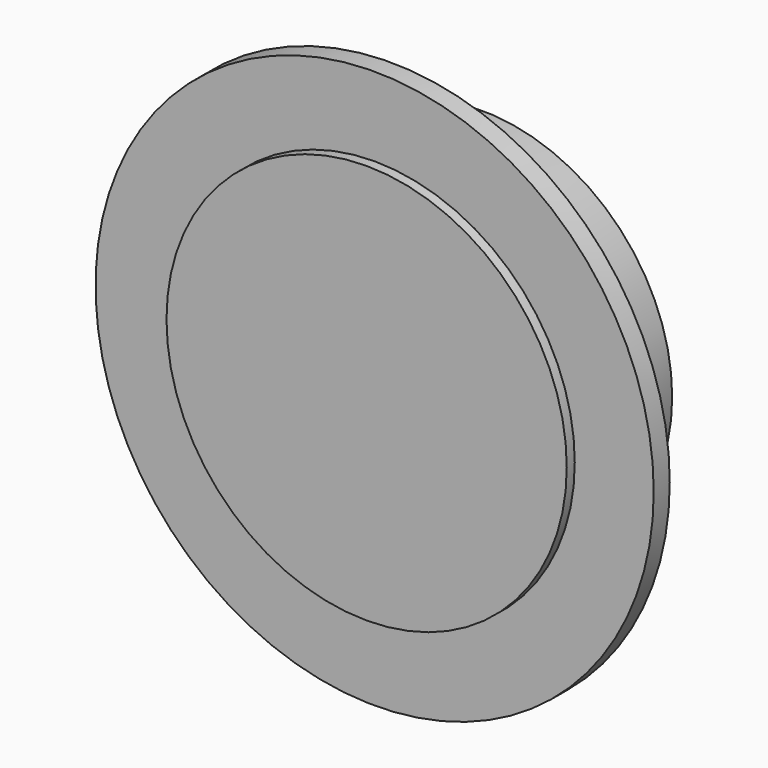
from build123d import *

# Parameters (mm, degrees)
F0_R      = 139.3871605201
F0_R_2    = 100
F1_DEPTH  = 10
F2_DEPTH  = 10
F0_R_3    = 99.95
F4_DEPTH  = 5
F3_R      = 100
F6_R      = 95
F8_R      = 40
F9_DEPTH  = 10
F10_R     = 22.575
F11_DEPTH = 5


# Not quite as in the source:
# - a feature names something its author has since deleted; it is built from what else it names


with BuildPart() as f1:
    # F0 (on Front) → F1 (new body)
    with BuildSketch(Plane.XZ):
        Circle(F0_R)
        Circle(F0_R_2, mode=Mode.SUBTRACT)
    extrude(amount=-F1_DEPTH)


with BuildPart() as f2:
    # F0 (on Front) → F2 (new body)
    with BuildSketch(Plane.XZ):
        Circle(F0_R)
        Circle(F0_R_2, mode=Mode.SUBTRACT)
    extrude(amount=-F2_DEPTH)


with BuildPart() as f4:
    # F0 (on Front) → F4 (new body)
    with BuildSketch(Plane.XZ):
        Circle(F0_R_3)
    extrude(amount=F4_DEPTH)

    # F3 (on face) → F7 section 0
    with BuildSketch(Plane.XZ):
        Circle(F3_R)
    # F6 (on offset) → F7 section 1
    with BuildSketch(Plane(origin=(0, 67, 0), x_dir=(-1, 0, 0), z_dir=(0, 1, 0))):
        Circle(F6_R)
    loft()

    # F8 (on offset) → F9 (cut)
    with BuildSketch(Plane(origin=(0, 67, 0), x_dir=(-1, 0, 0), z_dir=(0, 1, 0))):
        Circle(F8_R)
    extrude(amount=-F9_DEPTH, mode=Mode.SUBTRACT)

    # F10 (on face) → F11 (cut)
    with BuildSketch(Plane(origin=(0, 57, 0), x_dir=(-1, 0, 0), z_dir=(0, 1, 0))):
        Circle(F10_R)
    extrude(amount=-F11_DEPTH, mode=Mode.SUBTRACT)


solid = Compound([f1.part, f2.part, f4.part])
